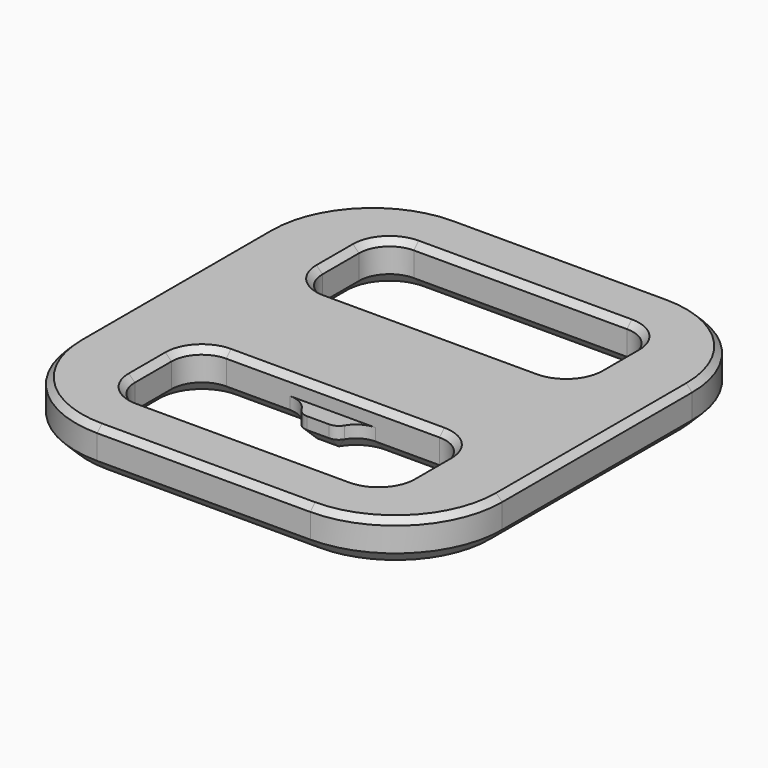
from build123d import *

# Parameters (mm, degrees)
F1_DEPTH = 7
F3_DEPTH = 4
F4_SIZE  = 1.99999
F8_SIZE  = 1


# Not quite as in the source:
# - a fillet or chamfer is up to 0.001 mm smaller than in the source, because OpenCascade refuses the exact size


with BuildPart() as f1:
    # F0 (on Top) → F1 (new body)
    with BuildSketch(Plane.XY):
        with BuildLine():
            Line((0, 10.5), (-17.5, 10.5))
            ThreePointArc((-17.5, 10.5), (-21.0355339059, 11.9644660941), (-22.5, 15.5))
            Line((-22.5, 15.5), (-22.5, 23))
            ThreePointArc((-22.5, 23), (-21.0355339059, 26.5355339059), (-17.5, 28))
            Line((-17.5, 28), (0, 28))
            Line((0, 28), (0, 37))
            Line((0, 37), (-17.5, 37))
            ThreePointArc((-17.5, 37), (-29.8743686708, 31.8743686708), (-35, 19.5))
            Line((-35, 19.5), (-35, 0))
            Line((-35, 0), (0, 0))
            Line((0, 0), (0, 10.5))
        make_face()
    extrude(amount=F1_DEPTH)

    # F2 (on Top) → F3 (join)
    with BuildSketch(Plane.XY):
        with BuildLine():
            Line((-7, 10.5), (0, 10.5))
            Line((0, 10.5), (0, 13.5))
            Line((0, 13.5), (-1.8038475773, 13.5))
            ThreePointArc((-1.8038475773, 13.5), (-2.8038475773, 13.2320508076), (-3.5358983849, 12.5))
            ThreePointArc((-3.5358983849, 12.5), (-5, 11.0358983849), (-7, 10.5))
        make_face()
    extrude(amount=F3_DEPTH)

    # F4 (size 2 in the source; OpenCascade refuses exactly that, so slightly less here)
    f4_edges = [f1.edges().sort_by_distance(p)[0] for p in [
        (-0.901924, 13.5, 0),
        (-35, 9.75, 0),
    ]]
    chamfer(f4_edges, length=F4_SIZE)

    # F6: F1 across face


with BuildPart() as f1_1:
    add(f1.part)
    add(f1.part.mirror(Plane(origin=(0, 6.0384247014, 3.3522948458), x_dir=(0, 1, 0), z_dir=(1, 0, 0))))

    # F7: F1 across face


with BuildPart() as f1_2:
    add(f1_1.part)
    add(f1_1.part.mirror(Plane(origin=(0, 0, 3.5233194082), x_dir=(1, 0, 0), z_dir=(0, -1, 0))))

    # F8
    f8_edges = [f1_2.edges().sort_by_distance(p)[0] for p in [
        (29.874369, 31.874369, 7),
        (0, 37, 7),
        (-29.874369, 31.874369, 7),
        (-35, 0, 7),
        (-29.874369, -31.874369, 7),
        (0, -37, 7),
        (29.874369, -31.874369, 7),
        (35, 0, 7),
        (-21.035534, 11.964466, 7),
        (-22.5, 19.25, 7),
        (-21.035534, 26.535534, 7),
        (0, 28, 7),
        (21.035534, 26.535534, 7),
        (22.5, 19.25, 7),
        (21.035534, 11.964466, 7),
        (0, 10.5, 7),
        (0, -10.5, 7),
        (21.035534, -11.964466, 7),
        (22.5, -19.25, 7),
        (21.035534, -26.535534, 7),
        (0, -28, 7),
        (-21.035534, -26.535534, 7),
        (-22.5, -19.25, 7),
        (-21.035534, -11.964466, 7),
    ]]
    chamfer(f8_edges, length=F8_SIZE)


solid = f1_2.part
